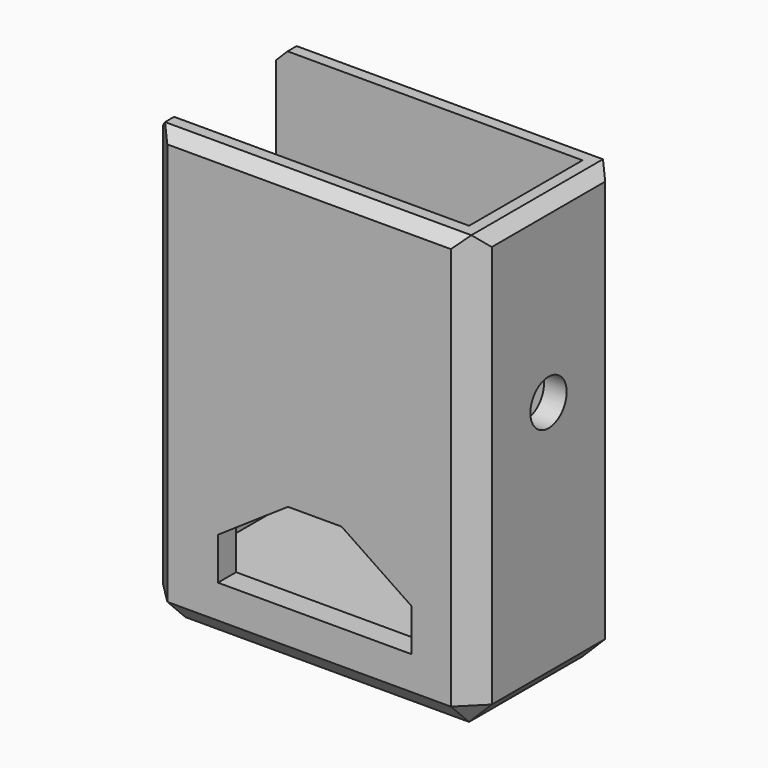
from build123d import *

# Parameters (mm, degrees)
F0_W      = 29
F0_H      = 16.5
F1_DEPTH  = 38.5
F2_T      = -2
F3_DEPTH  = 2.25
F4_SIZE   = 2
F5_SIZE   = 0.99999
F7_DEPTH  = 16.501
F9_DEPTH  = 2
F10_R     = 2
F11_DEPTH = 2.001
F12_W     = 5.538
F12_H     = 5.533
F14_W     = 5.538
F14_H     = 4.583


# Not quite as in the source:
# - a fillet or chamfer is up to 0.001 mm smaller than in the source, because OpenCascade refuses the exact size


with BuildPart() as f1:
    # F0 (on Top) → F1 (new body)
    with BuildSketch(Plane.XY):
        with Locations((14.5, 8.25)):
            Rectangle(F0_W, F0_H)
    extrude(amount=F1_DEPTH)

    # F2
    f2_openings = [f1.faces().sort_by_distance(p)[0] for p in [
        (14.5, 8.25, 38.5),
    ]]
    offset(amount=F2_T, openings=f2_openings)

    # F3 (add): a face of the model
    f3_faces = [f1.faces().sort_by_distance(p)[0] for p in [
        (14.5, 8.25, 2),
    ]]
    extrude(f3_faces, amount=F3_DEPTH)

    # F4
    f4_edges = [f1.edges().sort_by_distance(p)[0] for p in [
        (29, 0, 19.25),
        (29, 16.5, 19.25),
        (0, 0, 19.25),
        (0, 16.5, 19.25),
        (14.5, 0, 0),
        (0, 8.25, 0),
        (14.5, 16.5, 0),
        (29, 8.25, 0),
    ]]
    chamfer(f4_edges, length=F4_SIZE)

    # F5 (size 1 in the source; OpenCascade refuses exactly that, so slightly less here)
    f5_edges = [f1.edges().sort_by_distance(p)[0] for p in [
        (14.5, 0, 38.5),
        (29, 8.25, 38.5),
        (14.5, 16.5, 38.5),
        (0, 8.25, 38.5),
    ]]
    chamfer(f5_edges, length=F5_SIZE)

    # F6 (on face) → F7 (cut, through all)
    with BuildSketch(Plane.XZ):
        Polygon((6.464, 8.664), (6.464, 4.94), (23.536, 4.94), (23.536, 8.664), (17.364, 12.834), (12.635, 12.834), align=None)
    extrude(amount=-F7_DEPTH, mode=Mode.SUBTRACT)

    # F8 (on Right) → F9 (cut, through all)
    with BuildSketch(Plane.YZ):
        with BuildLine():
            Line((14.5, 38.5), (2, 38.5))
            Line((2, 38.5), (2, 28.5))
            ThreePointArc((2, 28.5), (8.25, 34.75), (14.5, 28.5))
            Line((14.5, 28.5), (14.5, 38.5))
        make_face()
        with BuildLine():
            ThreePointArc((14.5, 28.5), (8.25, 34.75), (2, 28.5))
            Line((2, 28.5), (14.5, 28.5))
        make_face()
        with BuildLine():
            Line((14.5, 28.5), (2, 28.5))
            ThreePointArc((2, 28.5), (2.8042583777, 25.4330148055), (5.0100474186, 23.1553571429))
            ThreePointArc((5.0100474186, 23.1553571429), (8.25, 26.15), (11.4899525814, 23.1553571429))
            ThreePointArc((11.4899525814, 23.1553571429), (13.6957416223, 25.4330148055), (14.5, 28.5))
        make_face()
        with BuildLine():
            ThreePointArc((11.4899525814, 23.1553571429), (8.25, 26.15), (5.0100474186, 23.1553571429))
            ThreePointArc((5.0100474186, 23.1553571429), (8.25, 22.25), (11.4899525814, 23.1553571429))
        make_face()
        with BuildLine():
            ThreePointArc((11.4899525814, 23.1553571429), (8.25, 22.25), (5.0100474186, 23.1553571429))
            ThreePointArc((5.0100474186, 23.1553571429), (8.122222634, 19.6525128261), (11.5, 22.9))
            ThreePointArc((11.5, 22.9), (11.4974871739, 23.027777366), (11.4899525814, 23.1553571429))
        make_face()
    extrude(amount=F9_DEPTH, mode=Mode.SUBTRACT)

    # F10 (on face) → F11 (cut, through all)
    with BuildSketch(Plane(origin=(27, 0, 0), x_dir=(0, -1, 0), z_dir=(-1, 0, 0))):
        with Locations((-8.25, 22.9)):
            Circle(F10_R)
    extrude(amount=-F11_DEPTH, mode=Mode.SUBTRACT)

    # F12 (on face) → F15 section 0
    with BuildSketch(Plane(origin=(0, 0, 0), x_dir=(0, -1, 0), z_dir=(-1, 0, 0))):
        with Locations((-8.25, 8.0385)):
            Rectangle(F12_W, F12_H)
    # F14 (on offset) → F15 section 1
    with BuildSketch(Plane(origin=(4.45, 0, 0), x_dir=(0, -1, 0), z_dir=(-1, 0, 0))):
        with Locations((-8.25, 8.5135)):
            Rectangle(F14_W, F14_H)
    loft(mode=Mode.SUBTRACT)


solid = f1.part
